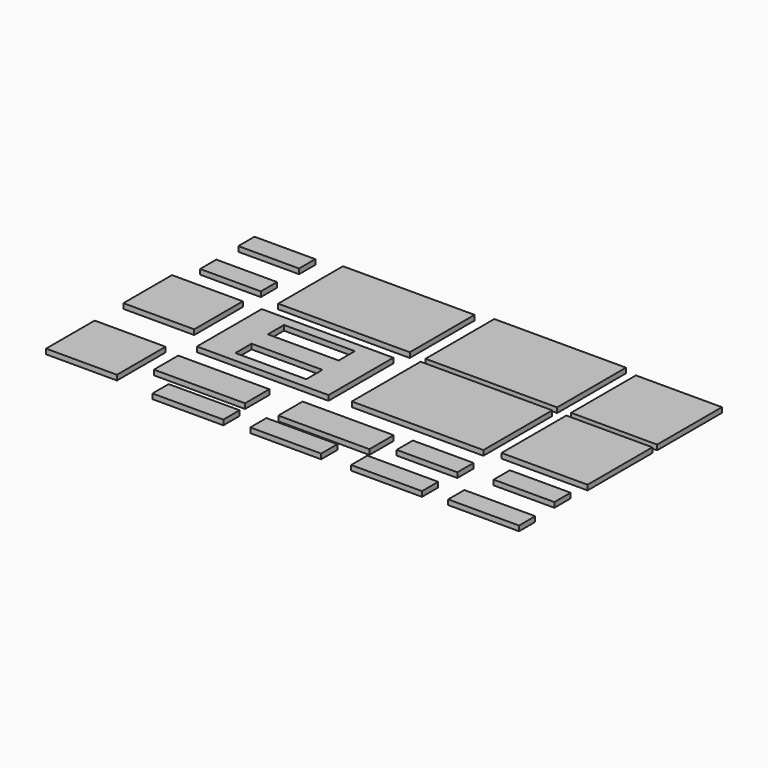
from build123d import *

# Parameters (mm, degrees)
F1_W      = 165.1
F1_H      = 107.95
F7_DEPTH  = 6.35
F2_W      = 165.1
F2_H      = 107.95
F3_W      = 107.95
F3_H      = 101.6
F4_W      = 107.95
F4_H      = 101.6
F5_W      = 165.1
F5_H      = 101.6
F6_W      = 165.1
F6_H      = 101.6
F8_W      = 88.9
F8_H      = 25.4
F9_DEPTH  = 6.351
F10_W     = 114.3
F10_H     = 38.1
F15_DEPTH = 6.35
F11_W     = 76.2
F11_H     = 25.4
F12_W     = 76.2
F12_H     = 25.4
F13_W     = 88.9
F13_H     = 76.2
F14_W     = 88.9
F14_H     = 25.4


# Not quite as in the source:
# - a variable given as a bare number and used for a length is read in inches; the dataset says mm whatever the document's units were


with BuildPart() as f7:
    # F1 (on Top) → F7 (new body)
    with BuildSketch(Plane.XY):
        with Locations((-54.9687035382, 61.838542049)):
            Rectangle(F1_W, F1_H)
    extrude(amount=F7_DEPTH)


with BuildPart() as f7b:
    # F2 (on Top) → F7, piece 2 (new body)
    with BuildSketch(Plane.XY):
        with Locations((-54.7917824507, -53.975)):
            Rectangle(F2_W, F2_H)
    extrude(amount=F7_DEPTH)


with BuildPart() as f7c:
    # F3 (on Top) → F7, piece 3 (new body)
    with BuildSketch(Plane.XY):
        with Locations((99.4075111032, 58.2500463382)):
            Rectangle(F3_W, F3_H)
    extrude(amount=F7_DEPTH)


with BuildPart() as f7d:
    # F4 (on Top) → F7, piece 4 (new body)
    with BuildSketch(Plane.XY):
        with Locations((99.3931097448, -50.8)):
            Rectangle(F4_W, F4_H)
    extrude(amount=F7_DEPTH)


with BuildPart() as f7e:
    # F5 (on Top) → F7, piece 5 (new body)
    with BuildSketch(Plane.XY):
        with Locations((-246.0931133747, -60.8584986448)):
            Rectangle(F5_W, F5_H)
    extrude(amount=F7_DEPTH)

    # F8 (on face) → F9 (cut, through all)
    with BuildSketch(Plane.XY.offset(6.35)):
        with Locations((-246.0931133747, -86.2584986448)):
            Rectangle(F8_W, F8_H)
        with Locations((-246.0931133747, -35.4584986448)):
            Rectangle(F8_W, F8_H)
    extrude(amount=-F9_DEPTH, mode=Mode.SUBTRACT)


with BuildPart() as f7f:
    # F6 (on Top) → F7, piece 6 (new body)
    with BuildSketch(Plane.XY):
        with Locations((-240.7411709428, 59.8363118468)):
            Rectangle(F6_W, F6_H)
    extrude(amount=F7_DEPTH)


with BuildPart() as f15:
    # F10 (on Top) → F15 (new body)
    with BuildSketch(Plane.XY):
        with Locations((-117.7062753201, -157.2435519218)):
            Rectangle(F10_W, F10_H)
    extrude(amount=F15_DEPTH)


with BuildPart() as f15b:
    # F10 (on Top) → F15, piece 2 (new body)
    with BuildSketch(Plane.XY):
        with Locations((-273.7219098568, -157.2435519218)):
            Rectangle(F10_W, F10_H)
    extrude(amount=F15_DEPTH)


with BuildPart() as f15c:
    # F11 (on Top) → F15, piece 3 (new body)
    with BuildSketch(Plane.XY):
        with Locations((-0.7997755945, -147.9919765472)):
            Rectangle(F11_W, F11_H)
    extrude(amount=F15_DEPTH)


with BuildPart() as f15d:
    # F11 (on Top) → F15, piece 4 (new body)
    with BuildSketch(Plane.XY):
        with Locations((112.8687295079, -137.962407279)):
            Rectangle(F11_W, F11_H)
    extrude(amount=F15_DEPTH)


with BuildPart() as f15e:
    # F12 (on Top) → F15, piece 5 (new body)
    with BuildSketch(Plane.XY):
        with Locations((-390.8388656616, 31.4260042876)):
            Rectangle(F12_W, F12_H)
    extrude(amount=F15_DEPTH)


with BuildPart() as f15f:
    # F12 (on Top) → F15, piece 6 (new body)
    with BuildSketch(Plane.XY):
        with Locations((-391.9532639027, 92.717849803)):
            Rectangle(F12_W, F12_H)
    extrude(amount=F15_DEPTH)


with BuildPart() as f15g:
    # F13 (on Top) → F15, piece 7 (new body)
    with BuildSketch(Plane.XY):
        with Locations((-397.8616445541, -46.812955761)):
            Rectangle(F13_W, F13_H)
    extrude(amount=F15_DEPTH)


with BuildPart() as f15h:
    # F13 (on Top) → F15, piece 8 (new body)
    with BuildSketch(Plane.XY):
        with Locations((-396.7472463131, -169.3966728687)):
            Rectangle(F13_W, F13_H)
    extrude(amount=F15_DEPTH)


with BuildPart() as f15i:
    # F14 (on face) → F15, piece 9 (new body)
    with BuildSketch(Plane.XY.offset(6.35)):
        with Locations((-1.5743746638, -210.3992934942)):
            Rectangle(F14_W, F14_H)
    extrude(amount=F15_DEPTH)


with BuildPart() as f15j:
    # F14 (on face) → F15, piece 10 (new body)
    with BuildSketch(Plane.XY.offset(6.35)):
        with Locations((-128.5148709297, -209.9128429174)):
            Rectangle(F14_W, F14_H)
    extrude(amount=F15_DEPTH)


with BuildPart() as f15k:
    # F14 (on face) → F15, piece 11 (new body)
    with BuildSketch(Plane.XY.offset(6.35)):
        with Locations((-248.337194252, -213.4719256639)):
            Rectangle(F14_W, F14_H)
    extrude(amount=F15_DEPTH)


with BuildPart() as f15l:
    # F14 (on face) → F15, piece 12 (new body)
    with BuildSketch(Plane.XY.offset(6.35)):
        with Locations((118.247956109, -208.0265666962)):
            Rectangle(F14_W, F14_H)
    extrude(amount=F15_DEPTH)


solid = Compound([f7.part, f7b.part, f7c.part, f7d.part, f7e.part, f7f.part, f15.part, f15b.part, f15c.part, f15d.part, f15e.part, f15f.part, f15g.part, f15h.part, f15i.part, f15j.part, f15k.part, f15l.part])
